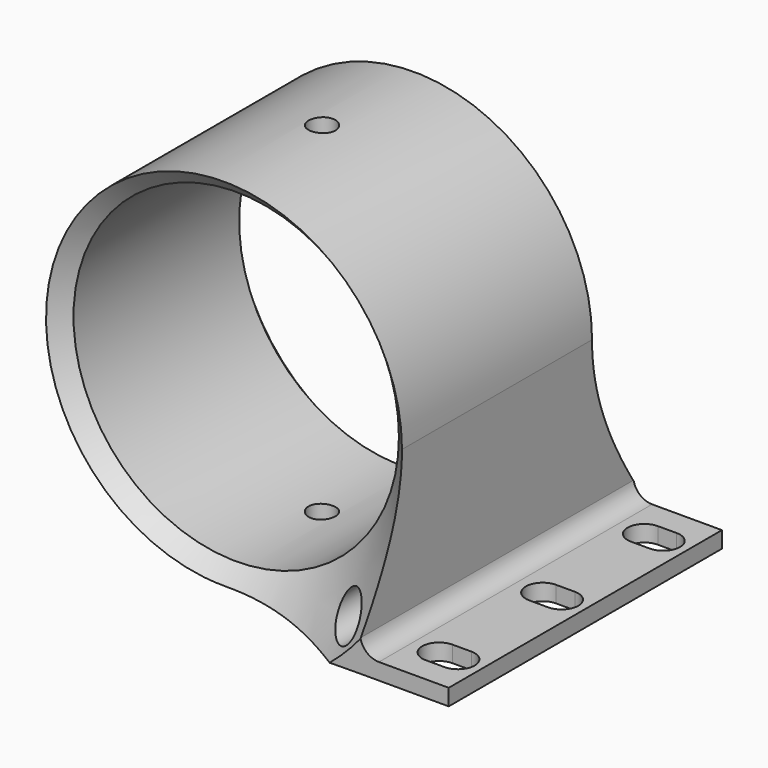
from build123d import *

# Parameters (mm, degrees)
F0_R     = 12.1031
F0_R_2   = 1.397
F1_DEPTH = 25.4
F4_DEPTH = 1.7
F8_R     = 1
F9_DEPTH = 27.8


# Not quite as in the source:
# - a fillet or chamfer that OpenCascade refuses, or shapes differently, is made with other operations: its cross-section is extruded or revolved along the edge and cut away or added


with BuildPart() as f1:
    # F0 (on Front) → F1 (new body)
    with BuildSketch(Plane.XZ):
        with BuildLine():
            ThreePointArc((0.1198459876, -13.2382072509), (9.403486197, -9.3187414184), (13.2387497249, 0))
            ThreePointArc((13.2387497249, 0), (-9.403486197, 9.3187414184), (0.1198459876, -13.2382072509))
        make_face()
        Circle(F0_R, mode=Mode.SUBTRACT)
        with BuildLine():
            Line((13.2387497249, -10.7690971345), (13.2387497249, 0))
            ThreePointArc((13.2387497249, 0), (9.403486197, -9.3187414184), (0.1198459876, -13.2382072509))
            Line((0.1198459876, -13.2382072509), (13.2387497249, -13.1194414571))
            Line((13.2387497249, -13.1194414571), (13.2387497249, -10.7690971345))
        make_face()
        with Locations((11.0441939905, -10.7448566705)):
            Circle(F0_R_2, mode=Mode.SUBTRACT)
        with BuildLine():
            ThreePointArc((14.6132539958, -11.9012827054), (13.7228739986, -11.5817927037), (13.2387497249, -10.7690971345))
            Line((13.2387497249, -10.7690971345), (13.2387497249, -13.1194414571))
            Line((13.2387497249, -13.1194414571), (19.8077764362, -13.1194414571))
            Line((19.8077764362, -13.1194414571), (19.8077764362, -11.9012827054))
            Line((19.8077764362, -11.9012827054), (14.6132539958, -11.9012827054))
        make_face()
    extrude(amount=F1_DEPTH)

    # F3 (on offset) → F4 (cut)
    with BuildSketch(Plane.XY.offset(-13.208)):
        with BuildLine():
            Line((16.5873928428, -4.4316952396), (17.9873928428, -4.4316952396))
            ThreePointArc((17.9873928428, -4.4316952396), (19.2373928428, -3.1816952396), (17.9873928428, -1.9316952396))
            Line((17.9873928428, -1.9316952396), (16.5873928428, -1.9316952396))
            ThreePointArc((16.5873928428, -1.9316952396), (15.3373928428, -3.1816952396), (16.5873928428, -4.4316952396))
        make_face()
        with BuildLine():
            Line((16.5873928428, -13.8912473619), (17.9873928428, -13.8912473619))
            ThreePointArc((17.9873928428, -13.8912473619), (19.2373928428, -12.6412473619), (17.9873928428, -11.3912473619))
            Line((17.9873928428, -11.3912473619), (16.5873928428, -11.3912473619))
            ThreePointArc((16.5873928428, -11.3912473619), (15.3373928428, -12.6412473619), (16.5873928428, -13.8912473619))
        make_face()
        with BuildLine():
            Line((16.5873928428, -23.5218666773), (17.9873928428, -23.5218666773))
            ThreePointArc((17.9873928428, -23.5218666773), (19.2373928428, -22.2718666773), (17.9873928428, -21.0218666773))
            Line((17.9873928428, -21.0218666773), (16.5873928428, -21.0218666773))
            ThreePointArc((16.5873928428, -21.0218666773), (15.3373928428, -22.2718666773), (16.5873928428, -23.5218666773))
        make_face()
    extrude(amount=F4_DEPTH, mode=Mode.SUBTRACT)

    # F5: chamfer of 5 on 1 edges, made by hand

    # F5_s1 → F5_t2 (revolve, cut)
    with BuildSketch(Plane.XY):
        Polygon((17.1031, -25.4), (12.1031, -20.4), (12.1031, -25.4), align=None)
    revolve(axis=Axis((0, -25.4, 0), (0, -1, 0)), mode=Mode.SUBTRACT)

    # F6: chamfer of 5 on 1 edges, made by hand

    # F6_s1 → F6_t2 (revolve, cut)
    with BuildSketch(Plane.XY):
        Polygon((17.1031, 0), (12.1031, -5), (12.1031, 0), align=None)
    revolve(axis=Axis((0, 0, 0), (0, -1, 0)), mode=Mode.SUBTRACT)

    # F8 (on offset) → F9 (cut)
    with BuildSketch(Plane.XY.offset(13.492)):
        with Locations((0, -12.424448505)):
            Circle(F8_R)
    extrude(amount=-F9_DEPTH, mode=Mode.SUBTRACT)


solid = f1.part
